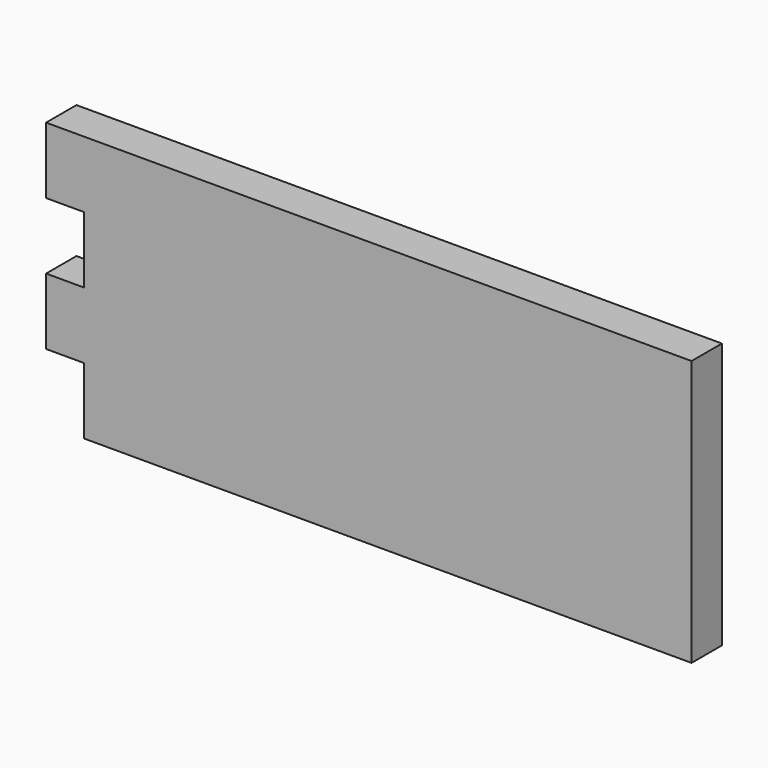
from build123d import *

# Parameters (mm, degrees)
F0_W     = 20
F0_H     = 35
F1_DEPTH = 20
F3_R     = 3.175
F4_DEPTH = 10


# Not quite as in the source:
# - a feature names something its author has since deleted; it is built from what else it names


with BuildPart() as f1:
    # F0 (on Front) → F1 (new body)
    with BuildSketch(Plane.XZ):
        with Locations((-160, 52.5)):
            Rectangle(F0_W, F0_H)
        with Locations((-160, -17.5)):
            Rectangle(F0_W, F0_H)
        Polygon((170, -70), (170, 70), (150, 70), (-150, 70), (-150, 35), (-150, 0), (-150, -35), (-150, -70), (150, -70), align=None)
    extrude(amount=-F1_DEPTH)

    # F3 (on face) → F4 (cut)
    with BuildSketch(Plane(origin=(0, 20, 0), x_dir=(-1, 0, 0), z_dir=(0, 1, 0))):
        with Locations((-160.0000113249, 35.0000448525)):
            Circle(F3_R)
        with Locations((-160.0000560284, 0)):
            Circle(F3_R)
        with Locations((-160.0000113249, -35.0000634789)):
            Circle(F3_R)
    extrude(amount=-F4_DEPTH, mode=Mode.SUBTRACT)


solid = f1.part
